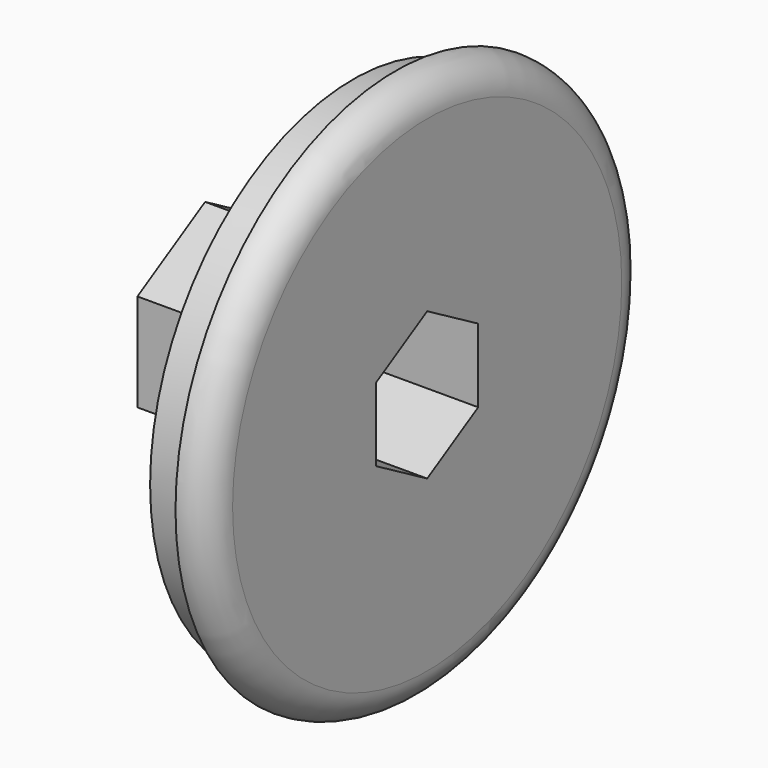
from build123d import *

# Parameters (mm, degrees)
F1_DEPTH = 14.2875
F2_R     = 20.6375
F3_DEPTH = 2.38125
F5_DEPTH = 9.525
F6_R     = 19.05
F6_R_2   = 17.4625
F7_DEPTH = 3.175
F8_R     = 2.38124


# Not quite as in the source:
# - a fillet or chamfer is up to 0.001 mm smaller than in the source, because OpenCascade refuses the exact size


with BuildPart() as f1:
    # F0 (on Right) → F1 (new body)
    with BuildSketch(Plane.YZ):
        Polygon((6.35, -3.6661742094), (6.35, 3.6661742094), (0, 7.3323484187), (-6.35, 3.6661742094), (-6.35, -3.6661742094), (0, -7.3323484187), align=None)
    extrude(amount=-F1_DEPTH)

    # F2 (on Right) → F3 (join)
    with BuildSketch(Plane.YZ):
        Circle(F2_R)
    extrude(amount=F3_DEPTH)

    # F4 (on face) → F5 (cut)
    with BuildSketch(Plane.YZ.offset(2.38125)):
        Polygon((4.7879, -2.7642953539), (4.7879, 2.7642953539), (0, 5.5285907077), (-4.7879, 2.7642953539), (-4.7879, -2.7642953539), (0, -5.5285907077), align=None)
    extrude(amount=-F5_DEPTH, mode=Mode.SUBTRACT)

    # F6 (on face) → F7 (join)
    with BuildSketch(Plane(origin=(0, 0, 0), x_dir=(0, -1, 0), z_dir=(-1, 0, 0))):
        Circle(F6_R)
        Circle(F6_R_2, mode=Mode.SUBTRACT)
    extrude(amount=F7_DEPTH)

    # F8 (radius 2.38125 in the source; OpenCascade refuses exactly that, so slightly less here)
    f8_edges = [f1.edges().sort_by_distance(p)[0] for p in [
        (2.38125, -20.6375, 0),
    ]]
    fillet(f8_edges, radius=F8_R)


solid = f1.part
